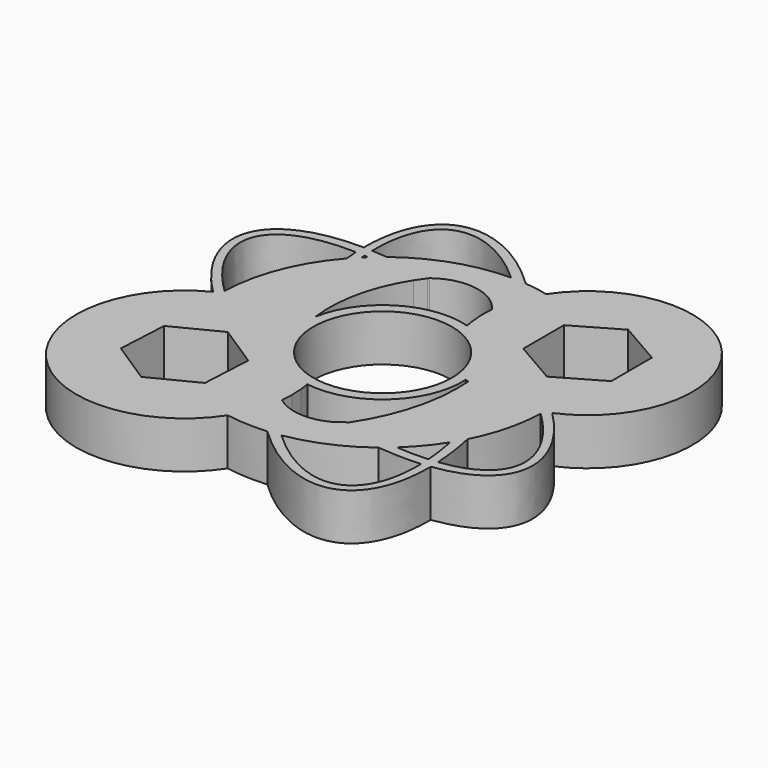
from build123d import *

# Parameters (mm, degrees)
F0_R     = 10.9
F1_DEPTH = 7.366
F2_DEPTH = 7.3


# Not quite as in the source:
# - a feature names something its author has since deleted; it is built from what else it names


with BuildPart() as f1:
    # F0 (on Top) → F1 (new body)
    with BuildSketch(Plane.XY):
        with BuildLine():
            ThreePointArc((26.3869951441, 0.3977309009), (32.4808941914, 26.1791281755), (6.0332161931, 24.6506061665))
            ThreePointArc((6.0332161931, 24.6506061665), (4.1919491801, 25.0295753875), (2.3276811495, 25.2712085677))
            add(Edge.make_bspline(
                [(2.3276811495, 25.2712085677), (-19.2874094687, 45.9525674234), (-19.2637930387, 20.3499966464)],
                knots=[2.2403697165, 2.2403697165, 2.2403697165, 3.8183770676, 3.8183770676, 3.8183770676], degree=2, weights=[1, 0.7045527085, 1]))
            add(Edge.make_bspline(
                [(-19.2637930387, 20.3499966464), (-47.4745392983, 20.7201874216), (-26.3374872786, -0.4473901376)],
                knots=[5.5212120323, 5.5212120323, 5.5212120323, 7.1314767866, 7.1314767866, 7.1314767866], degree=2, weights=[1, 0.6930158074, 1]))
            ThreePointArc((-26.3374872786, -0.4473901376), (-31.3645159289, -27.0254018787), (-4.3915569498, -24.9953257543))
            ThreePointArc((-4.3915569498, -24.9953257543), (-1.1617770215, -25.3515750233), (2.0870487223, -25.2922183614))
            add(Edge.make_bspline(
                [(2.0870487223, -25.2922183614), (23.8876265233, -46.1246356388), (23.6553453138, -20.1060092596)],
                knots=[5.3829862481, 5.3829862481, 5.3829862481, 6.9695320338, 6.9695320338, 6.9695320338], degree=2, weights=[1, 0.70151664, 1]))
            add(Edge.make_bspline(
                [(23.6553453138, -20.1060092596), (44.0507146815, -17.348583997), (26.3869951441, 0.3977309009)],
                knots=[2.5530868606, 2.5530868606, 2.5530868606, 3.9874437217, 3.9874437217, 3.9874437217], degree=2, weights=[1, 0.7536632337, 1]))
        make_face()
        Polygon((-25.7830432434, -19.2916921381), (-25.3610482326, -11.3065338088), (-18.2347007608, -7.6794130438), (-11.5303482997, -12.0374506081), (-11.9523433106, -20.0226089374), (-19.0786907824, -23.6497297024), align=None, mode=Mode.SUBTRACT)
        with BuildLine():
            add(Edge.make_bspline(
                [(4.0988276286, -25.0449933935), (22.8065750241, -42.4777662972), (22.273184435, -20.2544120195)],
                knots=[2.2989528501, 2.2989528501, 2.2989528501, 3.80327397, 3.80327397, 3.80327397], degree=2, weights=[1, 0.7302144408, 1]))
            ThreePointArc((4.0988276286, -25.0449933935), (10.0882623806, -23.2868856687), (15.4673710354, -20.1199531625))
            add(Edge.make_bspline(
                [(15.4673710354, -20.1199531625), (19.168293586, -20.5059961494), (22.273184435, -20.2544120195)],
                knots=[2.24559605, 2.24559605, 2.24559605, 2.4956246998, 2.4956246998, 2.4956246998], degree=2, weights=[1, 0.9921958812, 1]))
        make_face(mode=Mode.SUBTRACT)
        with BuildLine():
            ThreePointArc((13.0973297377, 0.4719694929), (12.250211614, -8.6875291134), (8.4943338963, -17.0843979587))
            ThreePointArc((8.4943338963, -17.0843979587), (8.4506142907, -17.1259954828), (8.4065764934, -17.1672560005))
            Line((8.4065764934, -17.1672560005), (6.5626807559, -18.4444562648))
            ThreePointArc((6.5626807559, -18.4444562648), (2.3036607791, -19.2340204791), (-1.7265882622, -17.6466467118))
            ThreePointArc((-1.7265882622, -17.6466467118), (-1.6433509144, -16.7149330714), (-1.6113495982, -15.7800562454))
            Line((-1.6113495982, -15.7800562454), (-1.703168006, -13.893961526))
            ThreePointArc((-1.703168006, -13.893961526), (-1.7965229638, -13.1562380977), (-1.921964033, -12.4232882065))
            ThreePointArc((-1.921964033, -12.4232882065), (8.4545317701, -9.3033826189), (12.5499699177, 0.7282105948))
            ThreePointArc((12.5499699177, 0.7282105948), (12.822477937, 0.5975867535), (13.0973297377, 0.4719694929))
        make_face(mode=Mode.SUBTRACT)
        with BuildLine():
            add(Edge.make_bspline(
                [(22.1982648609, -18.7297830777), (22.0198857543, -16.2878979371), (21.4659935183, -13.5374740732)],
                knots=[3.8658359172, 3.8658359172, 3.8658359172, 4.0607868306, 4.0607868306, 4.0607868306], degree=2, weights=[1, 0.9952530281, 1]))
            add(Edge.make_bspline(
                [(17.1943915625, -18.665609575), (19.8944697948, -18.8857918491), (22.1982648609, -18.7297830777)],
                knots=[2.3138858247, 2.3138858247, 2.3138858247, 2.5138145397, 2.5138145397, 2.5138145397], degree=2, weights=[1, 0.995007723, 1]))
            ThreePointArc((17.1943915625, -18.665609575), (19.4995073548, -16.2425766099), (21.4659935183, -13.5374740732))
        make_face(mode=Mode.SUBTRACT)
        with BuildLine():
            add(Edge.make_bspline(
                [(23.6063588648, -18.5939333245), (41.5891751739, -16.3069716763), (25.3708523837, -0.6098617321)],
                knots=[2.5770942426, 2.5770942426, 2.5770942426, 3.9692994825, 3.9692994825, 3.9692994825], degree=2, weights=[1, 0.7673471333, 1]))
            add(Edge.make_bspline(
                [(23.6063588648, -18.5939333245), (23.4251943066, -15.2931028921), (22.6063083156, -11.532862019)],
                knots=[0.7441073711, 0.7441073711, 0.7441073711, 0.9898388859, 0.9898388859, 0.9898388859], degree=2, weights=[1, 0.9924614934, 1]))
            ThreePointArc((22.6063083156, -11.532862019), (24.6024383143, -6.226725544), (25.3708523837, -0.6098617321))
        make_face(mode=Mode.SUBTRACT)
        with BuildLine():
            add(Edge.make_bspline(
                [(-19.2232891188, 18.7794363283), (-44.9204254271, 19.5311645939), (-25.3708523837, 0.6098617321)],
                knots=[5.5328321471, 5.5328321471, 5.5328321471, 7.110892136, 7.110892136, 7.110892136], degree=2, weights=[1, 0.704534031, 1]))
            add(Edge.make_bspline(
                [(-19.2232891188, 18.7794363283), (-19.174212229, 17.7890260339), (-19.0659640165, 16.749361126)],
                knots=[3.8787432601, 3.8787432601, 3.8787432601, 3.9531757638, 3.9531757638, 3.9531757638], degree=2, weights=[1, 0.9993075552, 1]))
            ThreePointArc((-19.0659640165, 16.749361126), (-23.638496634, 9.2343683536), (-25.3708523837, 0.6098617321))
        make_face(mode=Mode.SUBTRACT)
        Circle(F0_R, mode=Mode.SUBTRACT)
        with BuildLine():
            ThreePointArc((-7.9849172354, 18.8037133276), (-7.9052415466, 18.9080088866), (-7.8249572767, 19.0118367008))
            ThreePointArc((-7.8249572767, 19.0118367008), (-1.8454784635, 20.5463978113), (3.3972397674, 17.2871110442))
            ThreePointArc((3.3972397674, 17.2871110442), (3.3188714752, 16.1950105111), (3.3130174728, 15.100117414))
            Line((3.3130174728, 15.100117414), (3.4809340278, 13.1658658061))
            ThreePointArc((3.4809340278, 13.1658658061), (3.575746246, 12.5896030472), (3.6908678955, 12.017051626))
            ThreePointArc((3.6908678955, 12.017051626), (-6.5139282847, 10.7517800344), (-12.3602739173, 2.2925235645))
            ThreePointArc((-12.3602739173, 2.2925235645), (-12.0193354184, 10.0998742181), (-9.0219161309, 17.3169678785))
            Line((-9.0219161309, 17.3169678785), (-7.9849172354, 18.8037133276))
        make_face(mode=Mode.SUBTRACT)
        with BuildLine():
            add(Edge.make_bspline(
                [(-17.8041178815, 18.7108368888), (-17.7829783362, 18.4236749006), (-17.7565614947, 18.1316465301)],
                knots=[0.7250017486, 0.7250017486, 0.7250017486, 0.7479864856, 0.7479864856, 0.7479864856], degree=2, weights=[1, 0.9999339635, 1]))
            add(Edge.make_bspline(
                [(-17.1943915625, 18.665609575), (-17.501532613, 18.6906558918), (-17.8041178815, 18.7108368888)],
                knots=[5.4554784783, 5.4554784783, 5.4554784783, 5.4782959672, 5.4782959672, 5.4782959672], degree=2, weights=[1, 0.999934921, 1]))
            Line((-17.1943915625, 18.665609575), (-17.7565614947, 18.1316465301))
        make_face(mode=Mode.SUBTRACT)
        with BuildLine():
            add(Edge.make_bspline(
                [(-0.0676197326, 25.3780911335), (-18.3637567737, 42.0411758414), (-17.881633053, 20.3066459152)],
                knots=[5.4586444481, 5.4586444481, 5.4586444481, 6.9426654219, 6.9426654219, 6.9426654219], degree=2, weights=[1, 0.7371114202, 1]))
            ThreePointArc((-0.0676197326, 25.3780911335), (-8.2003651304, 24.0167877481), (-15.4673710354, 20.1199531625))
            add(Edge.make_bspline(
                [(-15.4673710354, 20.1199531625), (-16.7038989629, 20.248935309), (-17.881633053, 20.3066459152)],
                knots=[5.3871887036, 5.3871887036, 5.3871887036, 5.4711152671, 5.4711152671, 5.4711152671], degree=2, weights=[1, 0.9991196707, 1]))
        make_face(mode=Mode.SUBTRACT)
        Polygon((19.8266504146, 23.5555883415), (26.7516504146, 19.5574377274), (26.7516504146, 11.5611364991), (19.8266504146, 7.562985885), (12.9016504146, 11.5611364991), (12.9016504146, 19.5574377274), align=None, mode=Mode.SUBTRACT)
    extrude(amount=F1_DEPTH)

    # F0 (on Top) → F2 (join)
    with BuildSketch(Plane.XY):
        with BuildLine():
            ThreePointArc((26.3869951441, 0.3977309009), (32.4808941914, 26.1791281755), (6.0332161931, 24.6506061665))
            ThreePointArc((6.0332161931, 24.6506061665), (4.1919491801, 25.0295753875), (2.3276811495, 25.2712085677))
            add(Edge.make_bspline(
                [(2.3276811495, 25.2712085677), (-19.2874094687, 45.9525674234), (-19.2637930387, 20.3499966464)],
                knots=[2.2403697165, 2.2403697165, 2.2403697165, 3.8183770676, 3.8183770676, 3.8183770676], degree=2, weights=[1, 0.7045527085, 1]))
            add(Edge.make_bspline(
                [(-19.2637930387, 20.3499966464), (-47.4745392983, 20.7201874216), (-26.3374872786, -0.4473901376)],
                knots=[5.5212120323, 5.5212120323, 5.5212120323, 7.1314767866, 7.1314767866, 7.1314767866], degree=2, weights=[1, 0.6930158074, 1]))
            ThreePointArc((-26.3374872786, -0.4473901376), (-31.3645159289, -27.0254018787), (-4.3915569498, -24.9953257543))
            ThreePointArc((-4.3915569498, -24.9953257543), (-1.1617770215, -25.3515750233), (2.0870487223, -25.2922183614))
            add(Edge.make_bspline(
                [(2.0870487223, -25.2922183614), (23.8876265233, -46.1246356388), (23.6553453138, -20.1060092596)],
                knots=[5.3829862481, 5.3829862481, 5.3829862481, 6.9695320338, 6.9695320338, 6.9695320338], degree=2, weights=[1, 0.70151664, 1]))
            add(Edge.make_bspline(
                [(23.6553453138, -20.1060092596), (44.0507146815, -17.348583997), (26.3869951441, 0.3977309009)],
                knots=[2.5530868606, 2.5530868606, 2.5530868606, 3.9874437217, 3.9874437217, 3.9874437217], degree=2, weights=[1, 0.7536632337, 1]))
        make_face()
        Polygon((-25.7830432434, -19.2916921381), (-25.3610482326, -11.3065338088), (-18.2347007608, -7.6794130438), (-11.5303482997, -12.0374506081), (-11.9523433106, -20.0226089374), (-19.0786907824, -23.6497297024), align=None, mode=Mode.SUBTRACT)
        with BuildLine():
            add(Edge.make_bspline(
                [(4.0988276286, -25.0449933935), (22.8065750241, -42.4777662972), (22.273184435, -20.2544120195)],
                knots=[2.2989528501, 2.2989528501, 2.2989528501, 3.80327397, 3.80327397, 3.80327397], degree=2, weights=[1, 0.7302144408, 1]))
            ThreePointArc((4.0988276286, -25.0449933935), (10.0882623806, -23.2868856687), (15.4673710354, -20.1199531625))
            add(Edge.make_bspline(
                [(15.4673710354, -20.1199531625), (19.168293586, -20.5059961494), (22.273184435, -20.2544120195)],
                knots=[2.24559605, 2.24559605, 2.24559605, 2.4956246998, 2.4956246998, 2.4956246998], degree=2, weights=[1, 0.9921958812, 1]))
        make_face(mode=Mode.SUBTRACT)
        with BuildLine():
            ThreePointArc((13.0973297377, 0.4719694929), (12.250211614, -8.6875291134), (8.4943338963, -17.0843979587))
            ThreePointArc((8.4943338963, -17.0843979587), (8.4506142907, -17.1259954828), (8.4065764934, -17.1672560005))
            Line((8.4065764934, -17.1672560005), (6.5626807559, -18.4444562648))
            ThreePointArc((6.5626807559, -18.4444562648), (2.3036607791, -19.2340204791), (-1.7265882622, -17.6466467118))
            ThreePointArc((-1.7265882622, -17.6466467118), (-1.6433509144, -16.7149330714), (-1.6113495982, -15.7800562454))
            Line((-1.6113495982, -15.7800562454), (-1.703168006, -13.893961526))
            ThreePointArc((-1.703168006, -13.893961526), (-1.7965229638, -13.1562380977), (-1.921964033, -12.4232882065))
            ThreePointArc((-1.921964033, -12.4232882065), (8.4545317701, -9.3033826189), (12.5499699177, 0.7282105948))
            ThreePointArc((12.5499699177, 0.7282105948), (12.822477937, 0.5975867535), (13.0973297377, 0.4719694929))
        make_face(mode=Mode.SUBTRACT)
        with BuildLine():
            add(Edge.make_bspline(
                [(22.1982648609, -18.7297830777), (22.0198857543, -16.2878979371), (21.4659935183, -13.5374740732)],
                knots=[3.8658359172, 3.8658359172, 3.8658359172, 4.0607868306, 4.0607868306, 4.0607868306], degree=2, weights=[1, 0.9952530281, 1]))
            add(Edge.make_bspline(
                [(17.1943915625, -18.665609575), (19.8944697948, -18.8857918491), (22.1982648609, -18.7297830777)],
                knots=[2.3138858247, 2.3138858247, 2.3138858247, 2.5138145397, 2.5138145397, 2.5138145397], degree=2, weights=[1, 0.995007723, 1]))
            ThreePointArc((17.1943915625, -18.665609575), (19.4995073548, -16.2425766099), (21.4659935183, -13.5374740732))
        make_face(mode=Mode.SUBTRACT)
        with BuildLine():
            add(Edge.make_bspline(
                [(23.6063588648, -18.5939333245), (41.5891751739, -16.3069716763), (25.3708523837, -0.6098617321)],
                knots=[2.5770942426, 2.5770942426, 2.5770942426, 3.9692994825, 3.9692994825, 3.9692994825], degree=2, weights=[1, 0.7673471333, 1]))
            add(Edge.make_bspline(
                [(23.6063588648, -18.5939333245), (23.4251943066, -15.2931028921), (22.6063083156, -11.532862019)],
                knots=[0.7441073711, 0.7441073711, 0.7441073711, 0.9898388859, 0.9898388859, 0.9898388859], degree=2, weights=[1, 0.9924614934, 1]))
            ThreePointArc((22.6063083156, -11.532862019), (24.6024383143, -6.226725544), (25.3708523837, -0.6098617321))
        make_face(mode=Mode.SUBTRACT)
        with BuildLine():
            add(Edge.make_bspline(
                [(-19.2232891188, 18.7794363283), (-44.9204254271, 19.5311645939), (-25.3708523837, 0.6098617321)],
                knots=[5.5328321471, 5.5328321471, 5.5328321471, 7.110892136, 7.110892136, 7.110892136], degree=2, weights=[1, 0.704534031, 1]))
            add(Edge.make_bspline(
                [(-19.2232891188, 18.7794363283), (-19.174212229, 17.7890260339), (-19.0659640165, 16.749361126)],
                knots=[3.8787432601, 3.8787432601, 3.8787432601, 3.9531757638, 3.9531757638, 3.9531757638], degree=2, weights=[1, 0.9993075552, 1]))
            ThreePointArc((-19.0659640165, 16.749361126), (-23.638496634, 9.2343683536), (-25.3708523837, 0.6098617321))
        make_face(mode=Mode.SUBTRACT)
        Circle(F0_R, mode=Mode.SUBTRACT)
        with BuildLine():
            ThreePointArc((-7.9849172354, 18.8037133276), (-7.9052415466, 18.9080088866), (-7.8249572767, 19.0118367008))
            ThreePointArc((-7.8249572767, 19.0118367008), (-1.8454784635, 20.5463978113), (3.3972397674, 17.2871110442))
            ThreePointArc((3.3972397674, 17.2871110442), (3.3188714752, 16.1950105111), (3.3130174728, 15.100117414))
            Line((3.3130174728, 15.100117414), (3.4809340278, 13.1658658061))
            ThreePointArc((3.4809340278, 13.1658658061), (3.575746246, 12.5896030472), (3.6908678955, 12.017051626))
            ThreePointArc((3.6908678955, 12.017051626), (-6.5139282847, 10.7517800344), (-12.3602739173, 2.2925235645))
            ThreePointArc((-12.3602739173, 2.2925235645), (-12.0193354184, 10.0998742181), (-9.0219161309, 17.3169678785))
            Line((-9.0219161309, 17.3169678785), (-7.9849172354, 18.8037133276))
        make_face(mode=Mode.SUBTRACT)
        with BuildLine():
            add(Edge.make_bspline(
                [(-17.8041178815, 18.7108368888), (-17.7829783362, 18.4236749006), (-17.7565614947, 18.1316465301)],
                knots=[0.7250017486, 0.7250017486, 0.7250017486, 0.7479864856, 0.7479864856, 0.7479864856], degree=2, weights=[1, 0.9999339635, 1]))
            add(Edge.make_bspline(
                [(-17.1943915625, 18.665609575), (-17.501532613, 18.6906558918), (-17.8041178815, 18.7108368888)],
                knots=[5.4554784783, 5.4554784783, 5.4554784783, 5.4782959672, 5.4782959672, 5.4782959672], degree=2, weights=[1, 0.999934921, 1]))
            Line((-17.1943915625, 18.665609575), (-17.7565614947, 18.1316465301))
        make_face(mode=Mode.SUBTRACT)
        with BuildLine():
            add(Edge.make_bspline(
                [(-0.0676197326, 25.3780911335), (-18.3637567737, 42.0411758414), (-17.881633053, 20.3066459152)],
                knots=[5.4586444481, 5.4586444481, 5.4586444481, 6.9426654219, 6.9426654219, 6.9426654219], degree=2, weights=[1, 0.7371114202, 1]))
            ThreePointArc((-0.0676197326, 25.3780911335), (-8.2003651304, 24.0167877481), (-15.4673710354, 20.1199531625))
            add(Edge.make_bspline(
                [(-15.4673710354, 20.1199531625), (-16.7038989629, 20.248935309), (-17.881633053, 20.3066459152)],
                knots=[5.3871887036, 5.3871887036, 5.3871887036, 5.4711152671, 5.4711152671, 5.4711152671], degree=2, weights=[1, 0.9991196707, 1]))
        make_face(mode=Mode.SUBTRACT)
        Polygon((19.8266504146, 23.5555883415), (26.7516504146, 19.5574377274), (26.7516504146, 11.5611364991), (19.8266504146, 7.562985885), (12.9016504146, 11.5611364991), (12.9016504146, 19.5574377274), align=None, mode=Mode.SUBTRACT)
    extrude(amount=F2_DEPTH)


solid = f1.part
